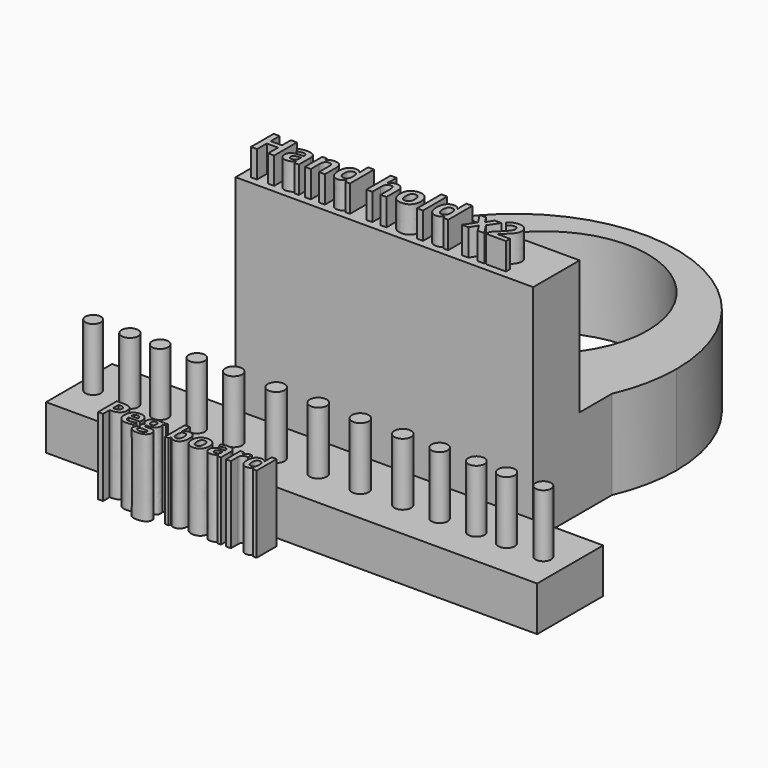
from build123d import *

# Parameters (mm, degrees)
F2_DEPTH      = 25.4
F3_R          = 29.4002099283
F4_DEPTH      = 56.134
F5_W          = 84.7290790428
F5_H          = 16.5136912838
F6_DEPTH      = 38.1
F7_W          = 139.7849097848
F7_H          = 23.4913118184
F8_DEPTH      = 12.7
F9_R          = 2.2065200044
F9_R_2        = 2.3719312557
F9_R_3        = 2.3024981392
F9_R_4        = 2.2907193351
F9_R_5        = 2.3946301528
F9_R_6        = 2.4199141052
F10_DEPTH     = 17.78
F11_TEXT_SIZE = 11.306323318
F12_DEPTH     = 7.62
F13_TEXT_SIZE = 9.3680909938
F14_DEPTH     = 21.844


# Not quite as in the source:
# - Text() gives the source's letters only with a copy of the font that has no kerning and outlines rounded to 1/6400 em; it was checked with that copy


with BuildPart() as f2:
    # F1 (on Top) → F2 (new body)
    with BuildSketch(Plane.XY):
        with BuildLine():
            ThreePointArc((42.2145798802, -0.7092366991), (45.0424739964, 8.2316942305), (45.9983477965, 17.5603348762))
            ThreePointArc((45.9983477965, 17.5603348762), (-8.9512926757, 62.6793149117), (-42.5144991626, 0))
            Line((-42.5144991626, 0), (42.2145798802, 0))
            Line((42.2145798802, 0), (42.2145798802, -0.7092366991))
        make_face()
        with BuildLine():
            Line((42.2145798802, 0), (-42.5144991626, 0))
            ThreePointArc((-42.5144991626, 0), (-0.3850221654, -28.4364015074), (42.2145798802, -0.7092366991))
            Line((42.2145798802, -0.7092366991), (42.2145798802, 0))
        make_face()
        with BuildLine():
            ThreePointArc((42.2145798802, -0.7092366991), (-0.3850221654, -28.4364015074), (-42.5144991626, 0))
            Line((-42.5144991626, 0), (-42.5144991626, -28.7245195359))
            Line((-42.5144991626, -28.7245195359), (42.2145798802, -28.7245195359))
            Line((42.2145798802, -28.7245195359), (42.2145798802, -0.7092366991))
        make_face()
    extrude(amount=F2_DEPTH)

    # F3 (on face) → F4 (cut)
    with BuildSketch(Plane.XY.offset(25.4)):
        with Locations((0, 28.0267577618)):
            Circle(F3_R)
    extrude(amount=-F4_DEPTH, mode=Mode.SUBTRACT)

    # F5 (on face) → F6 (join)
    with BuildSketch(Plane.XY.offset(25.4)):
        with Locations((-0.1499596412, -20.467673894)):
            Rectangle(F5_W, F5_H)
    extrude(amount=F6_DEPTH)

    # F11 (on face) → F12 (join)
    with BuildSketch(Plane.XY.offset(63.5)):
        with Locations((-40.8190563321, -26.6312360764)):
            Text('Hand hold x2', F11_TEXT_SIZE, font='Open Sans', font_style=FontStyle.BOLD, text_align=(TextAlign.LEFT, TextAlign.BOTTOM))
    extrude(amount=F12_DEPTH)


with BuildPart() as f8:
    # F7 (on Top) → F8 (new body)
    with BuildSketch(Plane.XY):
        with Locations((1.1629350483, -51.6343619674)):
            Rectangle(F7_W, F7_H)
    extrude(amount=F8_DEPTH)

    # F9 (on face) → F10 (join)
    with BuildSketch(Plane.XY.offset(12.7)):
        with Locations((-64.0777796507, -52.4484142661)):
            Circle(F9_R)
        with Locations((-53.6113530397, -52.4484142661)):
            Circle(F9_R_2)
        with Locations((-45.0056269765, -52.4484142661)):
            Circle(F9_R_3)
        with Locations((-34.5392003655, -52.4484142661)):
            Circle(F9_R_4)
        with Locations((-24.0727756172, -52.4484142661)):
            Circle(F9_R_5)
        with Locations((0, -52.4484142661)):
            Circle(F9_R_6)
        with Locations((-11.9782406837, -52.4484142661)):
            Circle(F9_R_5)
        with Locations((11.9782406837, -52.4484142661)):
            Circle(F9_R_5)
        with Locations((24.0727756172, -52.4484142661)):
            Circle(F9_R_5)
        with Locations((34.5392003655, -52.4484142661)):
            Circle(F9_R_4)
        with Locations((45.0056269765, -52.4484142661)):
            Circle(F9_R_3)
        with Locations((53.6113530397, -52.4484142661)):
            Circle(F9_R_2)
        with Locations((64.0777796507, -52.4484142661)):
            Circle(F9_R)
    extrude(amount=F10_DEPTH)


with BuildPart() as f14:
    # F13 (on Top) → F14 (new body)
    with BuildSketch(Plane.XY):
        with Locations((-46.5945425806, -73.6138522625)):
            Text('Peg board', F13_TEXT_SIZE, font='Open Sans', font_style=FontStyle.BOLD, text_align=(TextAlign.LEFT, TextAlign.BOTTOM))
    extrude(amount=F14_DEPTH)


solid = Compound([f2.part, f8.part, f14.part])
